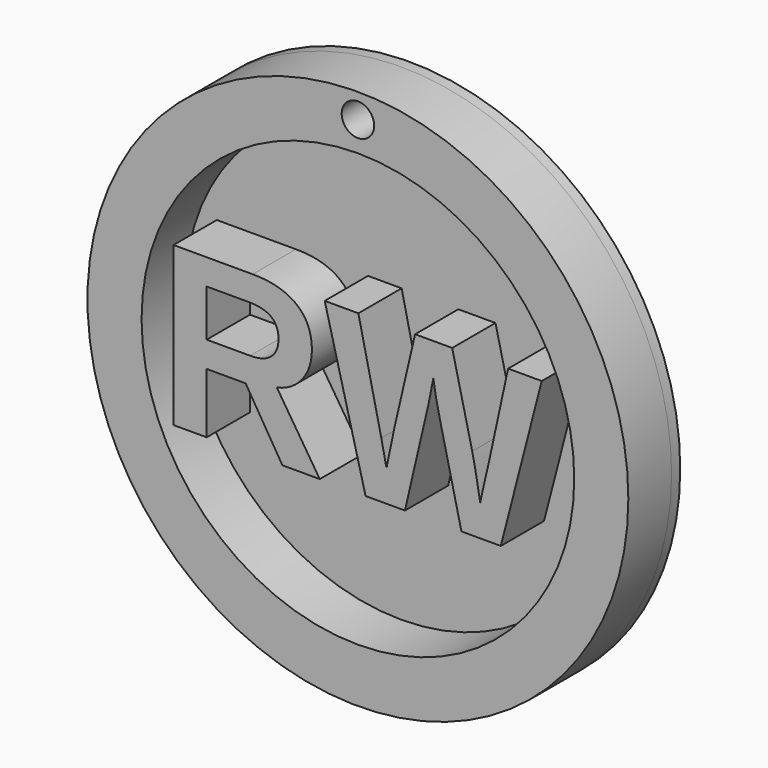
from build123d import *

# Parameters (mm, degrees)
F0_R         = 25
F0_R_2       = 20
F0_R_3       = 1.5
F0_TEXT_SIZE = 21.3005450794
F1_DEPTH     = 5
F2_R         = 25
F3_DEPTH     = 1


# Not quite as in the source:
# - Text() gives the source's letters only with a copy of the font that has no kerning and outlines rounded to 1/6400 em; it was checked with that copy


with BuildPart() as f1:
    # F0 (on Front) → F1 (new body)
    with BuildSketch(Plane.XZ):
        Circle(F0_R)
        Circle(F0_R_2, mode=Mode.SUBTRACT)
        with Locations((0, 22.7264445275)):
            Circle(F0_R_3, mode=Mode.SUBTRACT)
        with Locations((-18.471566436, -7.6681962286)):
            Text('RW', F0_TEXT_SIZE, font='Arimo', font_style=FontStyle.BOLD, text_align=(TextAlign.LEFT, TextAlign.BOTTOM))
    extrude(amount=F1_DEPTH)


with BuildPart() as f3:
    # F2 (on Front) → F3 (new body)
    with BuildSketch(Plane.XZ):
        Circle(F2_R)
    extrude(amount=-F3_DEPTH)


solid = Compound([f1.part, f3.part])
